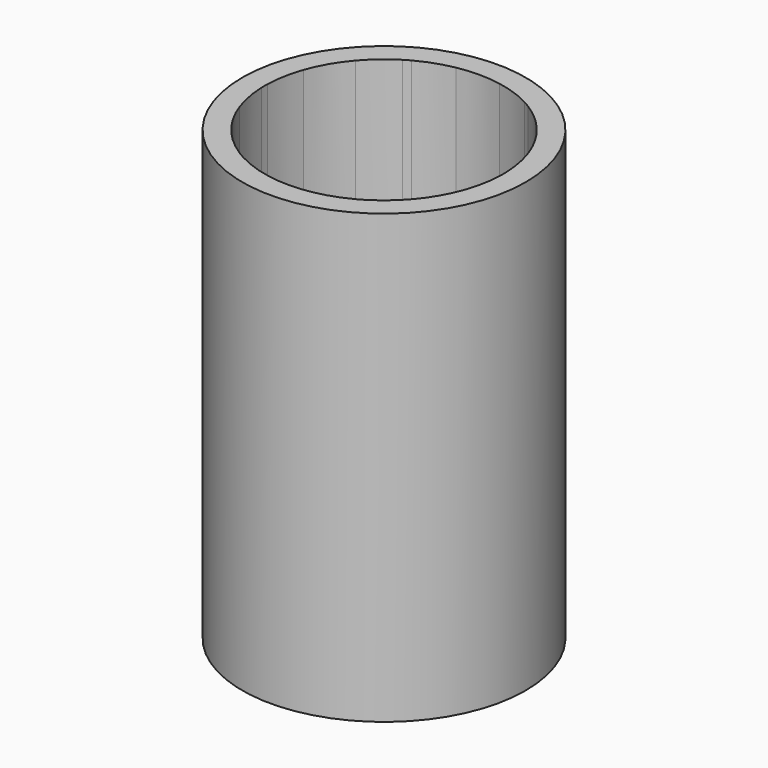
from build123d import *
from build123d import SkipClean  # not in build123d's __all__

# Parameters (mm, degrees)
F0_R     = 9.5
F1_DEPTH = 30
F2_R     = 8
F3_DEPTH = 12


with BuildPart() as f1:
    # F0 (on Top) → F1 (new body)
    with BuildSketch(Plane.XY):
        Circle(F0_R)
        with BuildLine():
            ThreePointArc((7.6873045768, 2.2148021003), (7.8289250313, 1.6455797926), (7.9284564034, 1.0675106838))
            Line((7.9284564034, 1.0675106838), (8.544783984, 0))
            Line((8.544783984, 0), (7.9284564034, -1.0675106838))
            ThreePointArc((7.9284564034, -1.0675106838), (7.8289250313, -1.6455797926), (7.6873045768, -2.2148021003))
            Line((7.6873045768, -2.2148021003), (8.544783984, -3.7))
            Line((8.544783984, -3.7), (7.476685986, -5.55))
            Line((7.476685986, -5.55), (5.7617271716, -5.55))
            ThreePointArc((5.7617271716, -5.55), (5.33957642, -5.9572580651), (4.8887195726, -6.3324893162))
            Line((4.8887195726, -6.3324893162), (4.272391992, -7.4))
            Line((4.272391992, -7.4), (3.0397368307, -7.4))
            ThreePointArc((3.0397368307, -7.4), (2.4893486113, -7.6028378578), (1.9255774052, -7.7648021003))
            Line((1.9255774052, -7.7648021003), (1.068097998, -9.25))
            Line((1.068097998, -9.25), (-1.068097998, -9.25))
            Line((-1.068097998, -9.25), (-1.9255774052, -7.7648021003))
            ThreePointArc((-1.9255774052, -7.7648021003), (-2.4893486113, -7.6028378578), (-3.0397368307, -7.4))
            Line((-3.0397368307, -7.4), (-4.272391992, -7.4))
            Line((-4.272391992, -7.4), (-4.8887195726, -6.3324893162))
            ThreePointArc((-4.8887195726, -6.3324893162), (-5.33957642, -5.9572580651), (-5.7617271716, -5.55))
            Line((-5.7617271716, -5.55), (-7.476685986, -5.55))
            Line((-7.476685986, -5.55), (-8.544783984, -3.7))
            Line((-8.544783984, -3.7), (-7.6873045768, -2.2148021003))
            ThreePointArc((-7.6873045768, -2.2148021003), (-7.8289250313, -1.6455797926), (-7.9284564034, -1.0675106838))
            Line((-7.9284564034, -1.0675106838), (-8.544783984, 0))
            Line((-8.544783984, 0), (-7.9284564034, 1.0675106838))
            ThreePointArc((-7.9284564034, 1.0675106838), (-7.8289250313, 1.6455797926), (-7.6873045768, 2.2148021003))
            Line((-7.6873045768, 2.2148021003), (-8.544783984, 3.7))
            Line((-8.544783984, 3.7), (-7.476685986, 5.55))
            Line((-7.476685986, 5.55), (-5.7617271716, 5.55))
            ThreePointArc((-5.7617271716, 5.55), (-5.33957642, 5.9572580651), (-4.8887195726, 6.3324893162))
            Line((-4.8887195726, 6.3324893162), (-4.272391992, 7.4))
            Line((-4.272391992, 7.4), (-3.0397368307, 7.4))
            ThreePointArc((-3.0397368307, 7.4), (-2.4893486113, 7.6028378578), (-1.9255774052, 7.7648021003))
            Line((-1.9255774052, 7.7648021003), (-1.068097998, 9.25))
            Line((-1.068097998, 9.25), (1.068097998, 9.25))
            Line((1.068097998, 9.25), (1.9255774052, 7.7648021003))
            ThreePointArc((1.9255774052, 7.7648021003), (2.4893486113, 7.6028378578), (3.0397368307, 7.4))
            Line((3.0397368307, 7.4), (4.272391992, 7.4))
            Line((4.272391992, 7.4), (4.8887195726, 6.3324893162))
            ThreePointArc((4.8887195726, 6.3324893162), (5.33957642, 5.9572580651), (5.7617271716, 5.55))
            Line((5.7617271716, 5.55), (7.476685986, 5.55))
            Line((7.476685986, 5.55), (8.544783984, 3.7))
            Line((8.544783984, 3.7), (7.6873045768, 2.2148021003))
        make_face(mode=Mode.SUBTRACT)
        Polygon((-2.136195996, 0), (-1.068097998, 1.85), (-2.136195996, 3.7), (-4.272391992, 3.7), (-5.34048999, 1.85), (-4.272391992, 0), align=None)
        Polygon((-4.0703193978, 3.35), (-2.3382685902, 3.35), (-1.4722431864, 1.85), (-2.3382685902, 0.35), (-4.0703193978, 0.35), (-4.9363448016, 1.85), align=None, mode=Mode.SUBTRACT)
        Polygon((-2.136195996, -3.7), (-1.068097998, -1.85), (-2.136195996, 0), (-4.272391992, 0), (-5.34048999, -1.85), (-4.272391992, -3.7), align=None)
        Polygon((-4.9363448016, -1.85), (-4.0703193978, -0.35), (-2.3382685902, -0.35), (-1.4722431864, -1.85), (-2.3382685902, -3.35), (-4.0703193978, -3.35), align=None, mode=Mode.SUBTRACT)
        Polygon((1.068097998, -5.55), (2.136195996, -3.7), (1.068097998, -1.85), (-1.068097998, -1.85), (-2.136195996, -3.7), (-1.068097998, -5.55), align=None)
        Polygon((-0.8660254038, -5.2), (-1.7320508076, -3.7), (-0.8660254038, -2.2), (0.8660254038, -2.2), (1.7320508076, -3.7), (0.8660254038, -5.2), align=None, mode=Mode.SUBTRACT)
        Polygon((4.272391992, -3.7), (5.34048999, -1.85), (4.272391992, 0), (2.136195996, 0), (1.068097998, -1.85), (2.136195996, -3.7), align=None)
        Polygon((4.9363448016, -1.85), (4.0703193978, -3.35), (2.3382685902, -3.35), (1.4722431864, -1.85), (2.3382685902, -0.35), (4.0703193978, -0.35), align=None, mode=Mode.SUBTRACT)
        Polygon((4.272391992, 0), (5.34048999, 1.85), (4.272391992, 3.7), (2.136195996, 3.7), (1.068097998, 1.85), (2.136195996, 0), align=None)
        Polygon((4.0703193978, 3.35), (4.9363448016, 1.85), (4.0703193978, 0.35), (2.3382685902, 0.35), (1.4722431864, 1.85), (2.3382685902, 3.35), align=None, mode=Mode.SUBTRACT)
        Polygon((1.068097998, 1.85), (2.136195996, 3.7), (1.068097998, 5.55), (-1.068097998, 5.55), (-2.136195996, 3.7), (-1.068097998, 1.85), align=None)
        Polygon((0.8660254038, 5.2), (1.7320508076, 3.7), (0.8660254038, 2.2), (-0.8660254038, 2.2), (-1.7320508076, 3.7), (-0.8660254038, 5.2), align=None, mode=Mode.SUBTRACT)
        Polygon((1.068097998, -1.85), (2.136195996, 0), (1.068097998, 1.85), (-1.068097998, 1.85), (-2.136195996, 0), (-1.068097998, -1.85), align=None)
        Polygon((0.8660254038, 1.5), (1.7320508076, 0), (0.8660254038, -1.5), (-0.8660254038, -1.5), (-1.7320508076, 0), (-0.8660254038, 1.5), align=None, mode=Mode.SUBTRACT)
        with BuildLine():
            Line((-2.136195996, 3.7), (-1.068097998, 5.55))
            Line((-1.068097998, 5.55), (-2.136195996, 7.4))
            Line((-2.136195996, 7.4), (-3.0397368307, 7.4))
            ThreePointArc((-3.0397368307, 7.4), (-3.41495707, 7.2345053881), (-3.7812035121, 7.05))
            Line((-3.7812035121, 7.05), (-2.3382685902, 7.05))
            Line((-2.3382685902, 7.05), (-1.4722431864, 5.55))
            Line((-1.4722431864, 5.55), (-2.3382685902, 4.05))
            Line((-2.3382685902, 4.05), (-4.0703193978, 4.05))
            Line((-4.0703193978, 4.05), (-4.9363448016, 5.55))
            Line((-4.9363448016, 5.55), (-4.2148773406, 6.7996182984))
            ThreePointArc((-4.2148773406, 6.7996182984), (-4.5577869149, 6.5746922695), (-4.8887195726, 6.3324893162))
            Line((-4.8887195726, 6.3324893162), (-5.34048999, 5.55))
            Line((-5.34048999, 5.55), (-4.272391992, 3.7))
            Line((-4.272391992, 3.7), (-2.136195996, 3.7))
        make_face()
        with BuildLine():
            Line((-5.34048999, -1.85), (-4.272391992, 0))
            Line((-4.272391992, 0), (-5.34048999, 1.85))
            Line((-5.34048999, 1.85), (-7.476685986, 1.85))
            Line((-7.476685986, 1.85), (-7.9284564034, 1.0675106838))
            ThreePointArc((-7.9284564034, 1.0675106838), (-7.9727439849, 0.6598131186), (-7.9960808527, 0.2503817016))
            Line((-7.9960808527, 0.2503817016), (-7.2746133918, 1.5))
            Line((-7.2746133918, 1.5), (-5.5425625842, 1.5))
            Line((-5.5425625842, 1.5), (-4.6765371804, 0))
            Line((-4.6765371804, 0), (-5.5425625842, -1.5))
            Line((-5.5425625842, -1.5), (-7.2746133918, -1.5))
            Line((-7.2746133918, -1.5), (-7.9960808527, -0.2503817016))
            ThreePointArc((-7.9960808527, -0.2503817016), (-7.9727439849, -0.6598131186), (-7.9284564034, -1.0675106838))
            Line((-7.9284564034, -1.0675106838), (-7.476685986, -1.85))
            Line((-7.476685986, -1.85), (-5.34048999, -1.85))
        make_face()
        with BuildLine():
            Line((-2.136195996, -7.4), (-1.068097998, -5.55))
            Line((-1.068097998, -5.55), (-2.136195996, -3.7))
            Line((-2.136195996, -3.7), (-4.272391992, -3.7))
            Line((-4.272391992, -3.7), (-5.34048999, -5.55))
            Line((-5.34048999, -5.55), (-4.8887195726, -6.3324893162))
            ThreePointArc((-4.8887195726, -6.3324893162), (-4.5577869149, -6.5746922695), (-4.2148773406, -6.7996182984))
            Line((-4.2148773406, -6.7996182984), (-4.9363448016, -5.55))
            Line((-4.9363448016, -5.55), (-4.0703193978, -4.05))
            Line((-4.0703193978, -4.05), (-2.3382685902, -4.05))
            Line((-2.3382685902, -4.05), (-1.4722431864, -5.55))
            Line((-1.4722431864, -5.55), (-2.3382685902, -7.05))
            Line((-2.3382685902, -7.05), (-3.7812035121, -7.05))
            ThreePointArc((-3.7812035121, -7.05), (-3.41495707, -7.2345053881), (-3.0397368307, -7.4))
            Line((-3.0397368307, -7.4), (-2.136195996, -7.4))
        make_face()
        with BuildLine():
            Line((2.136195996, 3.7), (4.272391992, 3.7))
            Line((4.272391992, 3.7), (5.34048999, 5.55))
            Line((5.34048999, 5.55), (4.8887195726, 6.3324893162))
            ThreePointArc((4.8887195726, 6.3324893162), (4.5577869149, 6.5746922695), (4.2148773406, 6.7996182984))
            Line((4.2148773406, 6.7996182984), (4.9363448016, 5.55))
            Line((4.9363448016, 5.55), (4.0703193978, 4.05))
            Line((4.0703193978, 4.05), (2.3382685902, 4.05))
            Line((2.3382685902, 4.05), (1.4722431864, 5.55))
            Line((1.4722431864, 5.55), (2.3382685902, 7.05))
            Line((2.3382685902, 7.05), (3.7812035121, 7.05))
            ThreePointArc((3.7812035121, 7.05), (3.41495707, 7.2345053881), (3.0397368307, 7.4))
            Line((3.0397368307, 7.4), (2.136195996, 7.4))
            Line((2.136195996, 7.4), (1.068097998, 5.55))
            Line((1.068097998, 5.55), (2.136195996, 3.7))
        make_face()
        with BuildLine():
            Line((7.2746133918, 1.5), (7.9960808527, 0.2503817016))
            ThreePointArc((7.9960808527, 0.2503817016), (7.9727439849, 0.6598131186), (7.9284564034, 1.0675106838))
            Line((7.9284564034, 1.0675106838), (7.476685986, 1.85))
            Line((7.476685986, 1.85), (5.34048999, 1.85))
            Line((5.34048999, 1.85), (4.272391992, 0))
            Line((4.272391992, 0), (5.34048999, -1.85))
            Line((5.34048999, -1.85), (7.476685986, -1.85))
            Line((7.476685986, -1.85), (7.9284564034, -1.0675106838))
            ThreePointArc((7.9284564034, -1.0675106838), (7.9727439849, -0.6598131186), (7.9960808527, -0.2503817016))
            Line((7.9960808527, -0.2503817016), (7.2746133918, -1.5))
            Line((7.2746133918, -1.5), (5.5425625842, -1.5))
            Line((5.5425625842, -1.5), (4.6765371804, 0))
            Line((4.6765371804, 0), (5.5425625842, 1.5))
            Line((5.5425625842, 1.5), (7.2746133918, 1.5))
        make_face()
        with BuildLine():
            Line((5.34048999, -5.55), (4.272391992, -3.7))
            Line((4.272391992, -3.7), (2.136195996, -3.7))
            Line((2.136195996, -3.7), (1.068097998, -5.55))
            Line((1.068097998, -5.55), (2.136195996, -7.4))
            Line((2.136195996, -7.4), (3.0397368307, -7.4))
            ThreePointArc((3.0397368307, -7.4), (3.41495707, -7.2345053881), (3.7812035121, -7.05))
            Line((3.7812035121, -7.05), (2.3382685902, -7.05))
            Line((2.3382685902, -7.05), (1.4722431864, -5.55))
            Line((1.4722431864, -5.55), (2.3382685902, -4.05))
            Line((2.3382685902, -4.05), (4.0703193978, -4.05))
            Line((4.0703193978, -4.05), (4.9363448016, -5.55))
            Line((4.9363448016, -5.55), (4.2148773406, -6.7996182984))
            ThreePointArc((4.2148773406, -6.7996182984), (4.5577869149, -6.5746922695), (4.8887195726, -6.3324893162))
            Line((4.8887195726, -6.3324893162), (5.34048999, -5.55))
        make_face()
        with BuildLine():
            Line((-5.34048999, 1.85), (-4.272391992, 3.7))
            Line((-4.272391992, 3.7), (-5.34048999, 5.55))
            Line((-5.34048999, 5.55), (-5.7617271716, 5.55))
            ThreePointArc((-5.7617271716, 5.55), (-5.9231861605, 5.3773474602), (-6.0794736614, 5.2))
            Line((-6.0794736614, 5.2), (-5.5425625842, 5.2))
            Line((-5.5425625842, 5.2), (-4.6765371804, 3.7))
            Line((-4.6765371804, 3.7), (-5.5425625842, 2.2))
            Line((-5.5425625842, 2.2), (-7.2746133918, 2.2))
            Line((-7.2746133918, 2.2), (-7.5430689304, 2.6649786324))
            ThreePointArc((-7.5430689304, 2.6649786324), (-7.6185125858, 2.4409559562), (-7.6873045768, 2.2148021003))
            Line((-7.6873045768, 2.2148021003), (-7.476685986, 1.85))
            Line((-7.476685986, 1.85), (-5.34048999, 1.85))
        make_face()
        with BuildLine():
            Line((-5.34048999, -5.55), (-4.272391992, -3.7))
            Line((-4.272391992, -3.7), (-5.34048999, -1.85))
            Line((-5.34048999, -1.85), (-7.476685986, -1.85))
            Line((-7.476685986, -1.85), (-7.6873045768, -2.2148021003))
            ThreePointArc((-7.6873045768, -2.2148021003), (-7.6185125858, -2.4409559562), (-7.5430689304, -2.6649786324))
            Line((-7.5430689304, -2.6649786324), (-7.2746133918, -2.2))
            Line((-7.2746133918, -2.2), (-5.5425625842, -2.2))
            Line((-5.5425625842, -2.2), (-4.6765371804, -3.7))
            Line((-4.6765371804, -3.7), (-5.5425625842, -5.2))
            Line((-5.5425625842, -5.2), (-6.0794736614, -5.2))
            ThreePointArc((-6.0794736614, -5.2), (-5.9231861605, -5.3773474602), (-5.7617271716, -5.55))
            Line((-5.7617271716, -5.55), (-5.34048999, -5.55))
        make_face()
        with BuildLine():
            Line((-1.068097998, 5.55), (1.068097998, 5.55))
            Line((1.068097998, 5.55), (2.136195996, 7.4))
            Line((2.136195996, 7.4), (1.9255774052, 7.7648021003))
            ThreePointArc((1.9255774052, 7.7648021003), (1.6953264253, 7.8183034165), (1.463595269, 7.8649786324))
            Line((1.463595269, 7.8649786324), (1.7320508076, 7.4))
            Line((1.7320508076, 7.4), (0.8660254038, 5.9))
            Line((0.8660254038, 5.9), (-0.8660254038, 5.9))
            Line((-0.8660254038, 5.9), (-1.7320508076, 7.4))
            Line((-1.7320508076, 7.4), (-1.463595269, 7.8649786324))
            ThreePointArc((-1.463595269, 7.8649786324), (-1.6953264253, 7.8183034165), (-1.9255774052, 7.7648021003))
            Line((-1.9255774052, 7.7648021003), (-2.136195996, 7.4))
            Line((-2.136195996, 7.4), (-1.068097998, 5.55))
        make_face()
        with BuildLine():
            Line((7.476685986, 1.85), (7.6873045768, 2.2148021003))
            ThreePointArc((7.6873045768, 2.2148021003), (7.6185125858, 2.4409559562), (7.5430689304, 2.6649786324))
            Line((7.5430689304, 2.6649786324), (7.2746133918, 2.2))
            Line((7.2746133918, 2.2), (5.5425625842, 2.2))
            Line((5.5425625842, 2.2), (4.6765371804, 3.7))
            Line((4.6765371804, 3.7), (5.5425625842, 5.2))
            Line((5.5425625842, 5.2), (6.0794736614, 5.2))
            ThreePointArc((6.0794736614, 5.2), (5.9231861605, 5.3773474602), (5.7617271716, 5.55))
            Line((5.7617271716, 5.55), (5.34048999, 5.55))
            Line((5.34048999, 5.55), (4.272391992, 3.7))
            Line((4.272391992, 3.7), (5.34048999, 1.85))
            Line((5.34048999, 1.85), (7.476685986, 1.85))
        make_face()
        with BuildLine():
            ThreePointArc((7.5430689304, -2.6649786324), (7.6185125858, -2.4409559562), (7.6873045768, -2.2148021003))
            Line((7.6873045768, -2.2148021003), (7.476685986, -1.85))
            Line((7.476685986, -1.85), (5.34048999, -1.85))
            Line((5.34048999, -1.85), (4.272391992, -3.7))
            Line((4.272391992, -3.7), (5.34048999, -5.55))
            Line((5.34048999, -5.55), (5.7617271716, -5.55))
            ThreePointArc((5.7617271716, -5.55), (5.9231861605, -5.3773474602), (6.0794736614, -5.2))
            Line((6.0794736614, -5.2), (5.5425625842, -5.2))
            Line((5.5425625842, -5.2), (4.6765371804, -3.7))
            Line((4.6765371804, -3.7), (5.5425625842, -2.2))
            Line((5.5425625842, -2.2), (7.2746133918, -2.2))
            Line((7.2746133918, -2.2), (7.5430689304, -2.6649786324))
        make_face()
        with BuildLine():
            Line((2.136195996, -7.4), (1.068097998, -5.55))
            Line((1.068097998, -5.55), (-1.068097998, -5.55))
            Line((-1.068097998, -5.55), (-2.136195996, -7.4))
            Line((-2.136195996, -7.4), (-1.9255774052, -7.7648021003))
            ThreePointArc((-1.9255774052, -7.7648021003), (-1.6953264253, -7.8183034165), (-1.463595269, -7.8649786324))
            Line((-1.463595269, -7.8649786324), (-1.7320508076, -7.4))
            Line((-1.7320508076, -7.4), (-0.8660254038, -5.9))
            Line((-0.8660254038, -5.9), (0.8660254038, -5.9))
            Line((0.8660254038, -5.9), (1.7320508076, -7.4))
            Line((1.7320508076, -7.4), (1.463595269, -7.8649786324))
            ThreePointArc((1.463595269, -7.8649786324), (1.6953264253, -7.8183034165), (1.9255774052, -7.7648021003))
            Line((1.9255774052, -7.7648021003), (2.136195996, -7.4))
        make_face()
        with BuildLine():
            Line((-7.2746133918, -5.2), (-6.0794736614, -5.2))
            ThreePointArc((-6.0794736614, -5.2), (-6.9282032303, -4), (-7.5430689304, -2.6649786324))
            Line((-7.5430689304, -2.6649786324), (-8.1406387956, -3.7))
            Line((-8.1406387956, -3.7), (-7.2746133918, -5.2))
        make_face()
        with BuildLine():
            ThreePointArc((-7.5430689304, 2.6649786324), (-6.9282032303, 4), (-6.0794736614, 5.2))
            Line((-6.0794736614, 5.2), (-7.2746133918, 5.2))
            Line((-7.2746133918, 5.2), (-8.1406387956, 3.7))
            Line((-8.1406387956, 3.7), (-7.5430689304, 2.6649786324))
        make_face()
        with BuildLine():
            ThreePointArc((-1.463595269, 7.8649786324), (0, 8), (1.463595269, 7.8649786324))
            Line((1.463595269, 7.8649786324), (0.8660254038, 8.9))
            Line((0.8660254038, 8.9), (-0.8660254038, 8.9))
            Line((-0.8660254038, 8.9), (-1.463595269, 7.8649786324))
        make_face()
        with BuildLine():
            ThreePointArc((6.0794736614, 5.2), (6.9282032303, 4), (7.5430689304, 2.6649786324))
            Line((7.5430689304, 2.6649786324), (8.1406387956, 3.7))
            Line((8.1406387956, 3.7), (7.2746133918, 5.2))
            Line((7.2746133918, 5.2), (6.0794736614, 5.2))
        make_face()
        with BuildLine():
            Line((8.1406387956, -3.7), (7.5430689304, -2.6649786324))
            ThreePointArc((7.5430689304, -2.6649786324), (6.9282032303, -4), (6.0794736614, -5.2))
            Line((6.0794736614, -5.2), (7.2746133918, -5.2))
            Line((7.2746133918, -5.2), (8.1406387956, -3.7))
        make_face()
        with BuildLine():
            Line((0.8660254038, -8.9), (1.463595269, -7.8649786324))
            ThreePointArc((1.463595269, -7.8649786324), (0, -8), (-1.463595269, -7.8649786324))
            Line((-1.463595269, -7.8649786324), (-0.8660254038, -8.9))
            Line((-0.8660254038, -8.9), (0.8660254038, -8.9))
        make_face()
        with BuildLine():
            ThreePointArc((-6.0794736614, 5.2), (-5.9231861605, 5.3773474602), (-5.7617271716, 5.55))
            Line((-5.7617271716, 5.55), (-7.476685986, 5.55))
            Line((-7.476685986, 5.55), (-8.544783984, 3.7))
            Line((-8.544783984, 3.7), (-7.6873045768, 2.2148021003))
            ThreePointArc((-7.6873045768, 2.2148021003), (-7.6185125858, 2.4409559562), (-7.5430689304, 2.6649786324))
            Line((-7.5430689304, 2.6649786324), (-8.1406387956, 3.7))
            Line((-8.1406387956, 3.7), (-7.2746133918, 5.2))
            Line((-7.2746133918, 5.2), (-6.0794736614, 5.2))
        make_face()
        with BuildLine():
            Line((-7.476685986, -5.55), (-5.7617271716, -5.55))
            ThreePointArc((-5.7617271716, -5.55), (-5.9231861605, -5.3773474602), (-6.0794736614, -5.2))
            Line((-6.0794736614, -5.2), (-7.2746133918, -5.2))
            Line((-7.2746133918, -5.2), (-8.1406387956, -3.7))
            Line((-8.1406387956, -3.7), (-7.5430689304, -2.6649786324))
            ThreePointArc((-7.5430689304, -2.6649786324), (-7.6185125858, -2.4409559562), (-7.6873045768, -2.2148021003))
            Line((-7.6873045768, -2.2148021003), (-8.544783984, -3.7))
            Line((-8.544783984, -3.7), (-7.476685986, -5.55))
        make_face()
        with BuildLine():
            ThreePointArc((1.463595269, 7.8649786324), (1.6953264253, 7.8183034165), (1.9255774052, 7.7648021003))
            Line((1.9255774052, 7.7648021003), (1.068097998, 9.25))
            Line((1.068097998, 9.25), (-1.068097998, 9.25))
            Line((-1.068097998, 9.25), (-1.9255774052, 7.7648021003))
            ThreePointArc((-1.9255774052, 7.7648021003), (-1.6953264253, 7.8183034165), (-1.463595269, 7.8649786324))
            Line((-1.463595269, 7.8649786324), (-0.8660254038, 8.9))
            Line((-0.8660254038, 8.9), (0.8660254038, 8.9))
            Line((0.8660254038, 8.9), (1.463595269, 7.8649786324))
        make_face()
        with BuildLine():
            ThreePointArc((7.5430689304, 2.6649786324), (7.6185125858, 2.4409559562), (7.6873045768, 2.2148021003))
            Line((7.6873045768, 2.2148021003), (8.544783984, 3.7))
            Line((8.544783984, 3.7), (7.476685986, 5.55))
            Line((7.476685986, 5.55), (5.7617271716, 5.55))
            ThreePointArc((5.7617271716, 5.55), (5.9231861605, 5.3773474602), (6.0794736614, 5.2))
            Line((6.0794736614, 5.2), (7.2746133918, 5.2))
            Line((7.2746133918, 5.2), (8.1406387956, 3.7))
            Line((8.1406387956, 3.7), (7.5430689304, 2.6649786324))
        make_face()
        with BuildLine():
            Line((8.544783984, -3.7), (7.6873045768, -2.2148021003))
            ThreePointArc((7.6873045768, -2.2148021003), (7.6185125858, -2.4409559562), (7.5430689304, -2.6649786324))
            Line((7.5430689304, -2.6649786324), (8.1406387956, -3.7))
            Line((8.1406387956, -3.7), (7.2746133918, -5.2))
            Line((7.2746133918, -5.2), (6.0794736614, -5.2))
            ThreePointArc((6.0794736614, -5.2), (5.9231861605, -5.3773474602), (5.7617271716, -5.55))
            Line((5.7617271716, -5.55), (7.476685986, -5.55))
            Line((7.476685986, -5.55), (8.544783984, -3.7))
        make_face()
        with BuildLine():
            Line((1.068097998, -9.25), (1.9255774052, -7.7648021003))
            ThreePointArc((1.9255774052, -7.7648021003), (1.6953264253, -7.8183034165), (1.463595269, -7.8649786324))
            Line((1.463595269, -7.8649786324), (0.8660254038, -8.9))
            Line((0.8660254038, -8.9), (-0.8660254038, -8.9))
            Line((-0.8660254038, -8.9), (-1.463595269, -7.8649786324))
            ThreePointArc((-1.463595269, -7.8649786324), (-1.6953264253, -7.8183034165), (-1.9255774052, -7.7648021003))
            Line((-1.9255774052, -7.7648021003), (-1.068097998, -9.25))
            Line((-1.068097998, -9.25), (1.068097998, -9.25))
        make_face()
        with BuildLine():
            Line((-8.544783984, 0), (-7.9284564034, -1.0675106838))
            ThreePointArc((-7.9284564034, -1.0675106838), (-7.9727439849, -0.6598131186), (-7.9960808527, -0.2503817016))
            Line((-7.9960808527, -0.2503817016), (-8.1406387956, 0))
            Line((-8.1406387956, 0), (-7.9960808527, 0.2503817016))
            ThreePointArc((-7.9960808527, 0.2503817016), (-7.9727439849, 0.6598131186), (-7.9284564034, 1.0675106838))
            Line((-7.9284564034, 1.0675106838), (-8.544783984, 0))
        make_face()
        with BuildLine():
            Line((-4.272391992, -7.4), (-3.0397368307, -7.4))
            ThreePointArc((-3.0397368307, -7.4), (-3.41495707, -7.2345053881), (-3.7812035121, -7.05))
            Line((-3.7812035121, -7.05), (-4.0703193978, -7.05))
            Line((-4.0703193978, -7.05), (-4.2148773406, -6.7996182984))
            ThreePointArc((-4.2148773406, -6.7996182984), (-4.5577869149, -6.5746922695), (-4.8887195726, -6.3324893162))
            Line((-4.8887195726, -6.3324893162), (-4.272391992, -7.4))
        make_face()
        with BuildLine():
            ThreePointArc((4.2148773406, 6.7996182984), (4.5577869149, 6.5746922695), (4.8887195726, 6.3324893162))
            Line((4.8887195726, 6.3324893162), (4.272391992, 7.4))
            Line((4.272391992, 7.4), (3.0397368307, 7.4))
            ThreePointArc((3.0397368307, 7.4), (3.41495707, 7.2345053881), (3.7812035121, 7.05))
            Line((3.7812035121, 7.05), (4.0703193978, 7.05))
            Line((4.0703193978, 7.05), (4.2148773406, 6.7996182984))
        make_face()
        with BuildLine():
            ThreePointArc((7.9284564034, 1.0675106838), (7.9727439849, 0.6598131186), (7.9960808527, 0.2503817016))
            Line((7.9960808527, 0.2503817016), (8.1406387956, 0))
            Line((8.1406387956, 0), (7.9960808527, -0.2503817016))
            ThreePointArc((7.9960808527, -0.2503817016), (7.9727439849, -0.6598131186), (7.9284564034, -1.0675106838))
            Line((7.9284564034, -1.0675106838), (8.544783984, 0))
            Line((8.544783984, 0), (7.9284564034, 1.0675106838))
        make_face()
        with BuildLine():
            Line((4.272391992, -7.4), (4.8887195726, -6.3324893162))
            ThreePointArc((4.8887195726, -6.3324893162), (4.5577869149, -6.5746922695), (4.2148773406, -6.7996182984))
            Line((4.2148773406, -6.7996182984), (4.0703193978, -7.05))
            Line((4.0703193978, -7.05), (3.7812035121, -7.05))
            ThreePointArc((3.7812035121, -7.05), (3.41495707, -7.2345053881), (3.0397368307, -7.4))
            Line((3.0397368307, -7.4), (4.272391992, -7.4))
        make_face()
        with BuildLine():
            ThreePointArc((-3.7812035121, 7.05), (-3.41495707, 7.2345053881), (-3.0397368307, 7.4))
            Line((-3.0397368307, 7.4), (-4.272391992, 7.4))
            Line((-4.272391992, 7.4), (-4.8887195726, 6.3324893162))
            ThreePointArc((-4.8887195726, 6.3324893162), (-4.5577869149, 6.5746922695), (-4.2148773406, 6.7996182984))
            Line((-4.2148773406, 6.7996182984), (-4.0703193978, 7.05))
            Line((-4.0703193978, 7.05), (-3.7812035121, 7.05))
        make_face()
        with BuildLine():
            Line((-5.7617271716, 5.55), (-5.34048999, 5.55))
            Line((-5.34048999, 5.55), (-4.8887195726, 6.3324893162))
            ThreePointArc((-4.8887195726, 6.3324893162), (-5.33957642, 5.9572580651), (-5.7617271716, 5.55))
        make_face()
        with BuildLine():
            Line((-7.9284564034, 1.0675106838), (-7.476685986, 1.85))
            Line((-7.476685986, 1.85), (-7.6873045768, 2.2148021003))
            ThreePointArc((-7.6873045768, 2.2148021003), (-7.8289250313, 1.6455797926), (-7.9284564034, 1.0675106838))
        make_face()
        with BuildLine():
            Line((-7.6873045768, -2.2148021003), (-7.476685986, -1.85))
            Line((-7.476685986, -1.85), (-7.9284564034, -1.0675106838))
            ThreePointArc((-7.9284564034, -1.0675106838), (-7.8289250313, -1.6455797926), (-7.6873045768, -2.2148021003))
        make_face()
        with BuildLine():
            Line((-4.8887195726, -6.3324893162), (-5.34048999, -5.55))
            Line((-5.34048999, -5.55), (-5.7617271716, -5.55))
            ThreePointArc((-5.7617271716, -5.55), (-5.33957642, -5.9572580651), (-4.8887195726, -6.3324893162))
        make_face()
        with BuildLine():
            Line((-3.0397368307, 7.4), (-2.136195996, 7.4))
            Line((-2.136195996, 7.4), (-1.9255774052, 7.7648021003))
            ThreePointArc((-1.9255774052, 7.7648021003), (-2.4893486113, 7.6028378578), (-3.0397368307, 7.4))
        make_face()
        with BuildLine():
            Line((1.9255774052, 7.7648021003), (2.136195996, 7.4))
            Line((2.136195996, 7.4), (3.0397368307, 7.4))
            ThreePointArc((3.0397368307, 7.4), (2.4893486113, 7.6028378578), (1.9255774052, 7.7648021003))
        make_face()
        with BuildLine():
            Line((5.34048999, 5.55), (5.7617271716, 5.55))
            ThreePointArc((5.7617271716, 5.55), (5.33957642, 5.9572580651), (4.8887195726, 6.3324893162))
            Line((4.8887195726, 6.3324893162), (5.34048999, 5.55))
        make_face()
        with BuildLine():
            Line((7.476685986, 1.85), (7.9284564034, 1.0675106838))
            ThreePointArc((7.9284564034, 1.0675106838), (7.8289250313, 1.6455797926), (7.6873045768, 2.2148021003))
            Line((7.6873045768, 2.2148021003), (7.476685986, 1.85))
        make_face()
        with BuildLine():
            ThreePointArc((7.6873045768, -2.2148021003), (7.8289250313, -1.6455797926), (7.9284564034, -1.0675106838))
            Line((7.9284564034, -1.0675106838), (7.476685986, -1.85))
            Line((7.476685986, -1.85), (7.6873045768, -2.2148021003))
        make_face()
        with BuildLine():
            ThreePointArc((4.8887195726, -6.3324893162), (5.33957642, -5.9572580651), (5.7617271716, -5.55))
            Line((5.7617271716, -5.55), (5.34048999, -5.55))
            Line((5.34048999, -5.55), (4.8887195726, -6.3324893162))
        make_face()
        with BuildLine():
            Line((-1.9255774052, -7.7648021003), (-2.136195996, -7.4))
            Line((-2.136195996, -7.4), (-3.0397368307, -7.4))
            ThreePointArc((-3.0397368307, -7.4), (-2.4893486113, -7.6028378578), (-1.9255774052, -7.7648021003))
        make_face()
        with BuildLine():
            Line((3.0397368307, -7.4), (2.136195996, -7.4))
            Line((2.136195996, -7.4), (1.9255774052, -7.7648021003))
            ThreePointArc((1.9255774052, -7.7648021003), (2.4893486113, -7.6028378578), (3.0397368307, -7.4))
        make_face()
        with BuildLine():
            Line((4.0703193978, -7.05), (4.2148773406, -6.7996182984))
            ThreePointArc((4.2148773406, -6.7996182984), (4, -6.9282032303), (3.7812035121, -7.05))
            Line((3.7812035121, -7.05), (4.0703193978, -7.05))
        make_face()
        with BuildLine():
            Line((-8.1406387956, 0), (-7.9960808527, -0.2503817016))
            ThreePointArc((-7.9960808527, -0.2503817016), (-8, 0), (-7.9960808527, 0.2503817016))
            Line((-7.9960808527, 0.2503817016), (-8.1406387956, 0))
        make_face()
        with BuildLine():
            Line((-4.0703193978, -7.05), (-3.7812035121, -7.05))
            ThreePointArc((-3.7812035121, -7.05), (-4, -6.9282032303), (-4.2148773406, -6.7996182984))
            Line((-4.2148773406, -6.7996182984), (-4.0703193978, -7.05))
        make_face()
        with BuildLine():
            ThreePointArc((7.9960808527, 0.2503817016), (7.9990201532, 0.1252061862), (8, 0))
            ThreePointArc((8, 0), (7.9990201532, -0.1252061862), (7.9960808527, -0.2503817016))
            Line((7.9960808527, -0.2503817016), (8.1406387956, 0))
            Line((8.1406387956, 0), (7.9960808527, 0.2503817016))
        make_face()
        with BuildLine():
            ThreePointArc((3.7812035121, 7.05), (4, 6.9282032303), (4.2148773406, 6.7996182984))
            Line((4.2148773406, 6.7996182984), (4.0703193978, 7.05))
            Line((4.0703193978, 7.05), (3.7812035121, 7.05))
        make_face()
        with BuildLine():
            ThreePointArc((-4.2148773406, 6.7996182984), (-4, 6.9282032303), (-3.7812035121, 7.05))
            Line((-3.7812035121, 7.05), (-4.0703193978, 7.05))
            Line((-4.0703193978, 7.05), (-4.2148773406, 6.7996182984))
        make_face()
    extrude(amount=-F1_DEPTH)

    # F2 (on Top) → F3 (cut)
    with BuildSketch(Plane.XY):
        Circle(F2_R)
    with SkipClean():  # cleaning this boolean's faces spoils the solid; the shape is the same uncleaned
        extrude(amount=-F3_DEPTH, mode=Mode.SUBTRACT)


solid = f1.part
